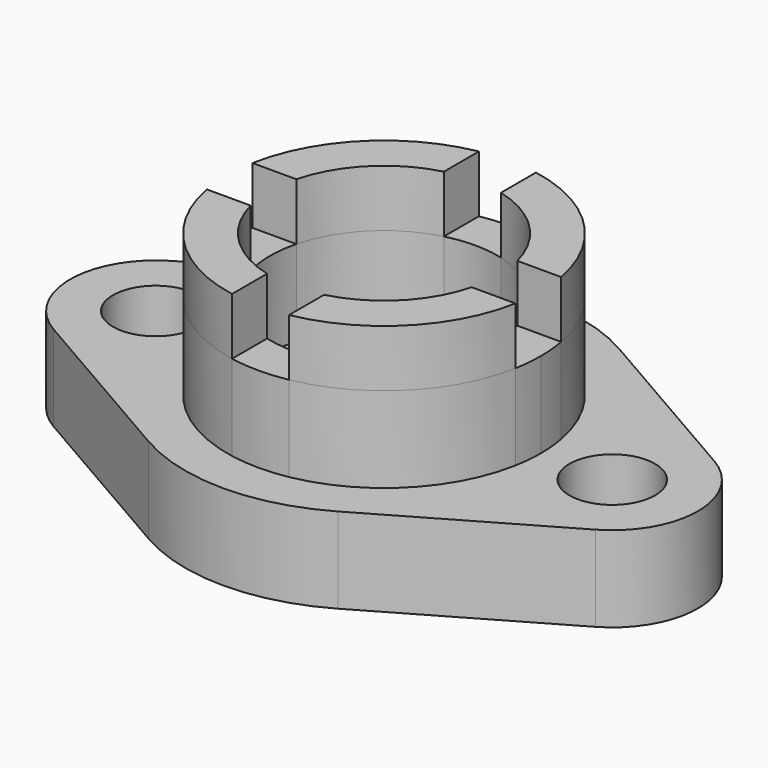
from build123d import *
from build123d import SkipClean  # not in build123d's __all__

# Parameters (mm, degrees)
F1_DEPTH = 38.1
F0_R     = 9.525
F2_DEPTH = 19.05
F0_R_2   = 12.7
F3_DEPTH = 19.05
F4_DEPTH = 50.8


with BuildPart() as f1:
    # F0 (on Top) → F1 (new body)
    with BuildSketch(Plane.XY):
        with BuildLine():
            ThreePointArc((6.35, 24.5934442484), (17.9605122421, 17.9605122421), (24.5934442484, 6.35))
            Line((24.5934442484, 6.35), (34.3428758988, 6.35))
            ThreePointArc((34.3428758988, 6.35), (24.6957043329, 24.6957043329), (6.35, 34.3428758988))
            Line((6.35, 34.3428758988), (6.35, 24.5934442484))
        make_face()
        with BuildLine():
            ThreePointArc((-6.35, 24.5934442484), (0, 25.4), (6.35, 24.5934442484))
            Line((6.35, 24.5934442484), (6.35, 34.3428758988))
            ThreePointArc((6.35, 34.3428758988), (0, 34.925), (-6.35, 34.3428758988))
            Line((-6.35, 34.3428758988), (-6.35, 24.5934442484))
        make_face()
        with BuildLine():
            ThreePointArc((-24.5934442484, 6.35), (-17.9605122421, 17.9605122421), (-6.35, 24.5934442484))
            Line((-6.35, 24.5934442484), (-6.35, 34.3428758988))
            ThreePointArc((-6.35, 34.3428758988), (-24.6957043329, 24.6957043329), (-34.3428758988, 6.35))
            Line((-34.3428758988, 6.35), (-24.5934442484, 6.35))
        make_face()
        with BuildLine():
            ThreePointArc((-24.5934442484, -6.35), (-25.4, 0), (-24.5934442484, 6.35))
            Line((-24.5934442484, 6.35), (-34.3428758988, 6.35))
            ThreePointArc((-34.3428758988, 6.35), (-34.925, 0), (-34.3428758988, -6.35))
            Line((-34.3428758988, -6.35), (-24.5934442484, -6.35))
        make_face()
        with BuildLine():
            Line((-6.35, -34.3428758988), (-6.35, -24.5934442484))
            ThreePointArc((-6.35, -24.5934442484), (-17.9605122421, -17.9605122421), (-24.5934442484, -6.35))
            Line((-24.5934442484, -6.35), (-34.3428758988, -6.35))
            ThreePointArc((-34.3428758988, -6.35), (-24.6957043329, -24.6957043329), (-6.35, -34.3428758988))
        make_face()
        with BuildLine():
            Line((6.35, -34.3428758988), (6.35, -24.5934442484))
            ThreePointArc((6.35, -24.5934442484), (0, -25.4), (-6.35, -24.5934442484))
            Line((-6.35, -24.5934442484), (-6.35, -34.3428758988))
            ThreePointArc((-6.35, -34.3428758988), (0, -34.925), (6.35, -34.3428758988))
        make_face()
        with BuildLine():
            Line((34.3428758988, -6.35), (24.5934442484, -6.35))
            ThreePointArc((24.5934442484, -6.35), (17.9605122421, -17.9605122421), (6.35, -24.5934442484))
            Line((6.35, -24.5934442484), (6.35, -34.3428758988))
            ThreePointArc((6.35, -34.3428758988), (24.6957043329, -24.6957043329), (34.3428758988, -6.35))
        make_face()
        with BuildLine():
            ThreePointArc((24.5934442484, 6.35), (25.1975542852, 3.2005090291), (25.4, 0))
            ThreePointArc((25.4, 0), (25.1975542852, -3.2005090291), (24.5934442484, -6.35))
            Line((24.5934442484, -6.35), (34.3428758988, -6.35))
            ThreePointArc((34.3428758988, -6.35), (34.7791644937, -3.1883133656), (34.925, 0))
            ThreePointArc((34.925, 0), (34.7791644937, 3.1883133656), (34.3428758988, 6.35))
            Line((34.3428758988, 6.35), (24.5934442484, 6.35))
        make_face()
    extrude(amount=F1_DEPTH)

    # F0 (on Top) → F2 (join)
    with BuildSketch(Plane.XY):
        with BuildLine():
            Line((-60.3174545175, -16.5021301071), (-21.0389726486, -39.1556398223))
            ThreePointArc((-21.0389726486, -39.1556398223), (0, -44.7878622326), (21.0389726486, -39.1556398223))
            Line((21.0389726486, -39.1556398223), (60.3174545175, -16.5021301071))
            ThreePointArc((60.3174545175, -16.5021301071), (69.8600459872, -0.008704331), (60.3325297632, 16.4934343301))
            Line((60.3325297632, 16.4934343301), (21.0389726486, 39.1556398223))
            ThreePointArc((21.0389726486, 39.1556398223), (0, 44.787862505), (-21.0389726486, 39.1556398223))
            Line((-21.0389726486, 39.1556398223), (-60.332536636, 16.4934343301))
            ThreePointArc((-60.332536636, 16.4934343301), (-69.8600525487, -0.0087063185), (-60.3174545175, -16.5021301071))
        make_face()
        with BuildLine():
            ThreePointArc((6.35, 34.3428758988), (24.6957043329, 24.6957043329), (34.3428758988, 6.35))
            ThreePointArc((34.3428758988, 6.35), (34.7791644937, 3.1883133656), (34.925, 0))
            ThreePointArc((34.925, 0), (34.7791644937, -3.1883133656), (34.3428758988, -6.35))
            ThreePointArc((34.3428758988, -6.35), (24.6957043329, -24.6957043329), (6.35, -34.3428758988))
            ThreePointArc((6.35, -34.3428758988), (0, -34.925), (-6.35, -34.3428758988))
            ThreePointArc((-6.35, -34.3428758988), (-24.6957043329, -24.6957043329), (-34.3428758988, -6.35))
            ThreePointArc((-34.3428758988, -6.35), (-34.925, 0), (-34.3428758988, 6.35))
            ThreePointArc((-34.3428758988, 6.35), (-24.6957043329, 24.6957043329), (-6.35, 34.3428758988))
            ThreePointArc((-6.35, 34.3428758988), (0, 34.925), (6.35, 34.3428758988))
        make_face(mode=Mode.SUBTRACT)
        with Locations((-50.7999965718, 5.9441e-06)):
            Circle(F0_R, mode=Mode.SUBTRACT)
        with Locations((50.7999931345, 3.9617e-06)):
            Circle(F0_R, mode=Mode.SUBTRACT)
    extrude(amount=F2_DEPTH)

    # F0 (on Top) → F3 (join)
    with BuildSketch(Plane.XY):
        with BuildLine():
            ThreePointArc((24.5934442484, -6.35), (25.1975542852, -3.2005090291), (25.4, 0))
            ThreePointArc((25.4, 0), (25.1975542852, 3.2005090291), (24.5934442484, 6.35))
            ThreePointArc((24.5934442484, 6.35), (17.9605122421, 17.9605122421), (6.35, 24.5934442484))
            ThreePointArc((6.35, 24.5934442484), (0, 25.4), (-6.35, 24.5934442484))
            ThreePointArc((-6.35, 24.5934442484), (-17.9605122421, 17.9605122421), (-24.5934442484, 6.35))
            ThreePointArc((-24.5934442484, 6.35), (-25.4, 0), (-24.5934442484, -6.35))
            ThreePointArc((-24.5934442484, -6.35), (-17.9605122421, -17.9605122421), (-6.35, -24.5934442484))
            ThreePointArc((-6.35, -24.5934442484), (0, -25.4), (6.35, -24.5934442484))
            ThreePointArc((6.35, -24.5934442484), (17.9605122421, -17.9605122421), (24.5934442484, -6.35))
        make_face()
        Circle(F0_R_2, mode=Mode.SUBTRACT)
    extrude(amount=F3_DEPTH)

    # F0 (on Top) → F4 (join)
    with BuildSketch(Plane.XY):
        with BuildLine():
            ThreePointArc((-24.5934442484, 6.35), (-17.9605122421, 17.9605122421), (-6.35, 24.5934442484))
            Line((-6.35, 24.5934442484), (-6.35, 34.3428758988))
            ThreePointArc((-6.35, 34.3428758988), (-24.6957043329, 24.6957043329), (-34.3428758988, 6.35))
            Line((-34.3428758988, 6.35), (-24.5934442484, 6.35))
        make_face()
        with BuildLine():
            ThreePointArc((6.35, 24.5934442484), (17.9605122421, 17.9605122421), (24.5934442484, 6.35))
            Line((24.5934442484, 6.35), (34.3428758988, 6.35))
            ThreePointArc((34.3428758988, 6.35), (24.6957043329, 24.6957043329), (6.35, 34.3428758988))
            Line((6.35, 34.3428758988), (6.35, 24.5934442484))
        make_face()
        with BuildLine():
            Line((34.3428758988, -6.35), (24.5934442484, -6.35))
            ThreePointArc((24.5934442484, -6.35), (17.9605122421, -17.9605122421), (6.35, -24.5934442484))
            Line((6.35, -24.5934442484), (6.35, -34.3428758988))
            ThreePointArc((6.35, -34.3428758988), (24.6957043329, -24.6957043329), (34.3428758988, -6.35))
        make_face()
        with BuildLine():
            Line((-6.35, -34.3428758988), (-6.35, -24.5934442484))
            ThreePointArc((-6.35, -24.5934442484), (-17.9605122421, -17.9605122421), (-24.5934442484, -6.35))
            Line((-24.5934442484, -6.35), (-34.3428758988, -6.35))
            ThreePointArc((-34.3428758988, -6.35), (-24.6957043329, -24.6957043329), (-6.35, -34.3428758988))
        make_face()
    with SkipClean():  # cleaning this boolean's faces spoils the solid; the shape is the same uncleaned
        extrude(amount=F4_DEPTH)


solid = f1.part
